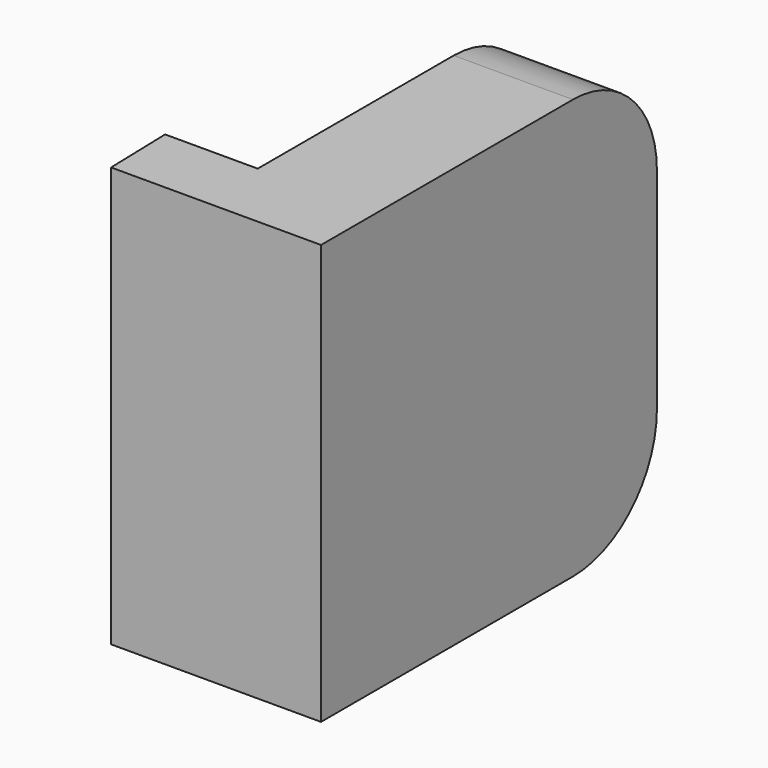
from build123d import *

# Parameters (mm, degrees)
F1_DEPTH = 76.2
F2_R     = 38.1


# Not quite as in the source:
# - ends of sketch curves that miss each other by under 0.0002 mm in the source are joined


with BuildPart() as f1:
    # F0 (on Top) → F1 (new body, symmetric)
    with BuildSketch(Plane.XY):
        Polygon((21.6444802228, 76.2), (-21.6444802228, 76.2), (-21.6444802228, -50.8097953513), (-55.2607951227, -50.8097953513), (-54.5555197772, -76.2), (-21.6444802228, -76.2), (21.6444802228, -76.2), align=None)
    extrude(amount=F1_DEPTH, both=True)

    # F2
    f2_edges = [f1.edges().sort_by_distance(p)[0] for p in [
        (0, 76.2, -76.2),
        (0, 76.2, 76.2),
    ]]
    fillet(f2_edges, radius=F2_R)


solid = f1.part
